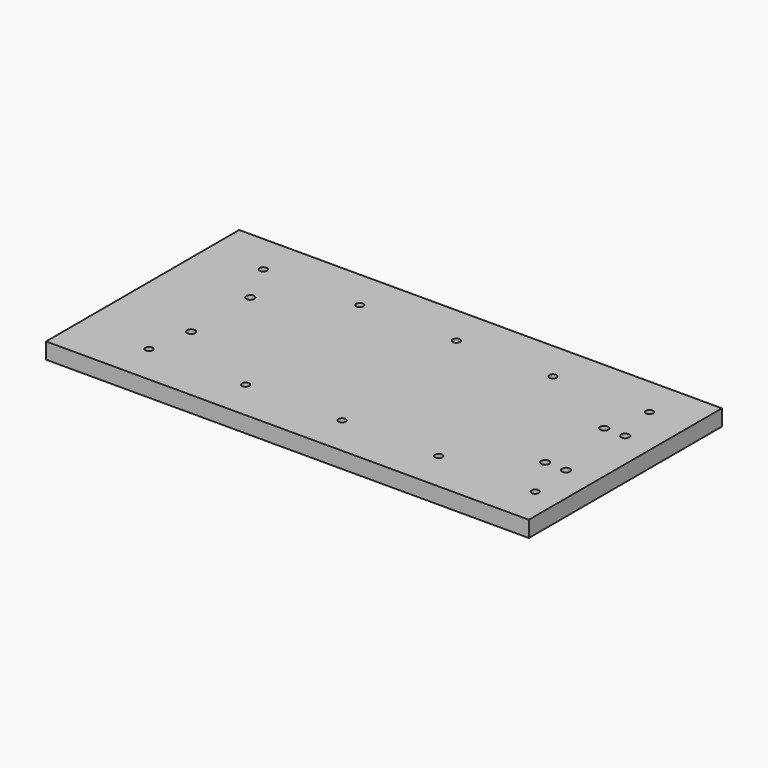
from build123d import *

# Parameters (mm, degrees)
F0_W     = 300
F0_H     = 150
F1_DEPTH = 10
F2_D     = 4.5
F4_D     = 5


# Not quite as in the source:
# - a feature names something its author has since deleted; it is built from what else it names


with BuildPart() as f1:
    # F0 (on Top) → F1 (new body)
    with BuildSketch(Plane.XY):
        Rectangle(F0_W, F0_H)
    extrude(amount=F1_DEPTH)

    # F2 (through all)
    with Locations(Plane(origin=(0, 0, 0), x_dir=(1, 0, 0), z_dir=(0, 0, -1))):
        with Locations((125, -50), (65, -50), (-55, -50), (-115, -50), (5, -50), (134, 50), (74, 50), (14, 50), (-46, 50), (-106, 50)):
            Hole(F2_D / 2)

    # F4 (through all)
    with Locations(Plane.XY.offset(10)):
        with Locations((118.5, 23), (131.5, 23), (131.5, -23), (118.5, -23), (-101.5, 23), (-101.5, -23)):
            Hole(F4_D / 2)


solid = f1.part
